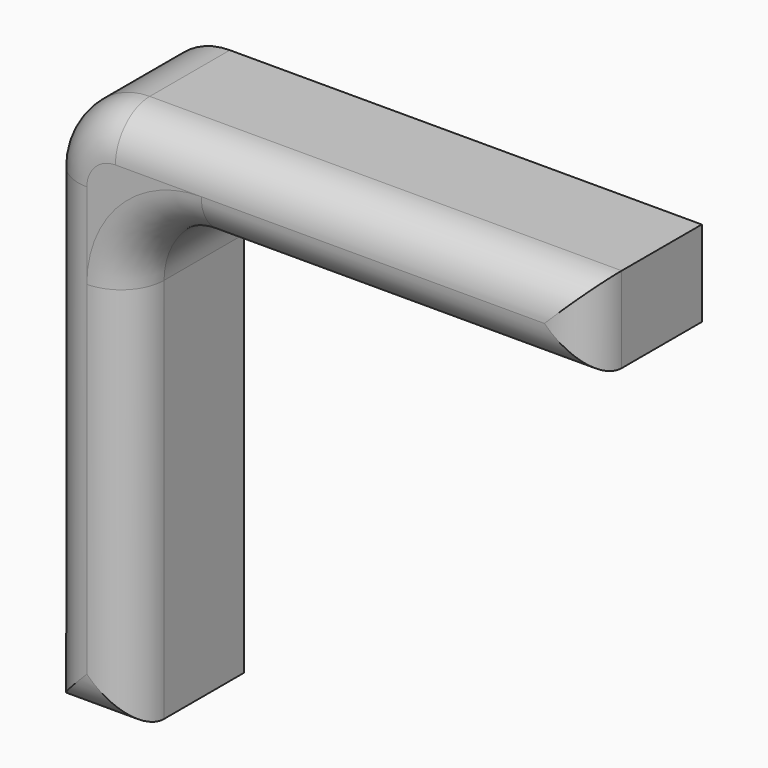
from build123d import *

# Parameters (mm, degrees)
F1_DEPTH      = 10
F3_DEPTH      = 10
F3_DEPTH_BACK = 8
F4_R          = 5
F5_R          = 2.99999


# Not quite as in the source:
# - a fillet or chamfer is up to 0.001 mm smaller than in the source, because OpenCascade refuses the exact size


with BuildPart() as f1:
    # F0 (on Front) → F1 (new body)
    with BuildSketch(Plane.XZ):
        Polygon((38, 0), (0, 0), (0, -38), (6, -38), (6, -6), (38, -6), align=None)
    extrude(amount=F1_DEPTH)

    # F2 (on Front) → F3 (cut, two sides)
    with BuildSketch(Plane.XZ) as f3_sk:
        Polygon((36, -2), (2, -2), (2, -36), (4, -36), (4, -4), (36, -4), align=None)
    extrude(amount=-F3_DEPTH, mode=Mode.SUBTRACT)
    extrude(f3_sk.sketch, amount=F3_DEPTH_BACK, mode=Mode.SUBTRACT)

    # F4
    f4_edges = [f1.edges().sort_by_distance(p)[0] for p in [
        (0, -5, 0),
        (4, -4, -4),
        (2, -4, -2),
        (6, -5, -6),
    ]]
    fillet(f4_edges, radius=F4_R)

    # F5 (radius 3 in the source; OpenCascade refuses exactly that, so slightly less here)
    f5_edges = [f1.edges().sort_by_distance(p)[0] for p in [
        (3, -10, -38),
        (6, -10, -24.5),
        (21.5, -10, 0),
        (38, -10, -3),
    ]]
    fillet(f5_edges, radius=F5_R)


solid = f1.part
